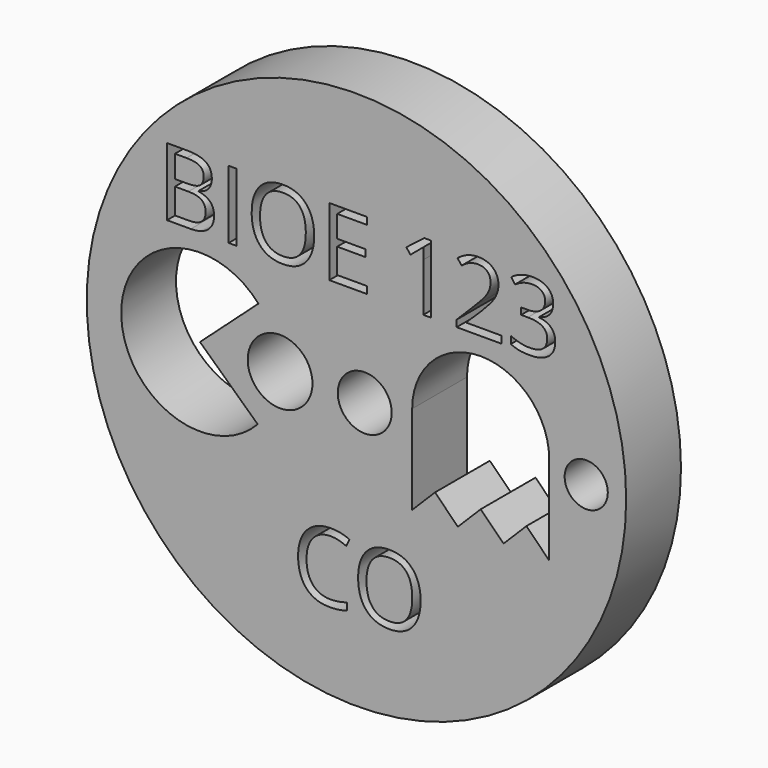
from build123d import *

# Parameters (mm, degrees)
F0_R         = 25
F1_DEPTH     = 6.35
F2_R         = 3
F2_R_2       = 2.5
F2_R_3       = 2
F2_TEXT_SIZE = 8.8194444444
F3_DEPTH     = 25.4


# Not quite as in the source:
# - Text() gives the source's letters only with a copy of the font that has no kerning and outlines rounded to 1/6400 em; it was checked with that copy


with BuildPart() as f1:
    # F0 (on Front) → F1 (new body)
    with BuildSketch(Plane.XZ):
        Circle(F0_R)
    extrude(amount=F1_DEPTH)

    # F2 (on face) → F3 (cut)
    with BuildSketch(Plane.XZ.offset(6.35)):
        with BuildLine():
            Line((-14.503664148, 0), (-9.0826506039, 4.8927618382))
            ThreePointArc((-9.0826506039, 4.8927618382), (-21.8059565626, 0.055061248), (-9.1570482839, -4.9739526588))
            Line((-9.1570482839, -4.9739526588), (-14.503664148, 0))
        make_face()
        with Locations((-7.077938877, 0)):
            Circle(F2_R)
        with BuildLine():
            ThreePointArc((17.86520852, 0.9525), (11.51520852, 7.3025), (5.16520852, 0.9525))
            Line((5.16520852, 0.9525), (5.16520852, -7.3025))
            Line((5.16520852, -7.3025), (7.2818751867, -5.1858333333))
            Line((7.2818751867, -5.1858333333), (9.3985418533, -7.3025))
            Line((9.3985418533, -7.3025), (11.51520852, -5.1858333333))
            Line((11.51520852, -5.1858333333), (13.6318751867, -7.3025))
            Line((13.6318751867, -7.3025), (15.7485418533, -5.1858333333))
            Line((15.7485418533, -5.1858333333), (17.86520852, -7.3025))
            Line((17.86520852, -7.3025), (17.86520852, 0.9525))
        make_face()
        with Locations((0.7674464141, 0)):
            Circle(F2_R_2)
        with Locations((21.2963800877, 0)):
            Circle(F2_R_3)
        with Locations((-18.4236816406, 8.9444242582)):
            Text('BIOE 123', F2_TEXT_SIZE, font='Open Sans', text_align=(TextAlign.LEFT, TextAlign.BOTTOM))
        with Locations((-5.9476128472, -17.6382309675)):
            Text('CO', F2_TEXT_SIZE, font='Open Sans', text_align=(TextAlign.LEFT, TextAlign.BOTTOM))
    extrude(amount=-F3_DEPTH, mode=Mode.SUBTRACT)


solid = f1.part
